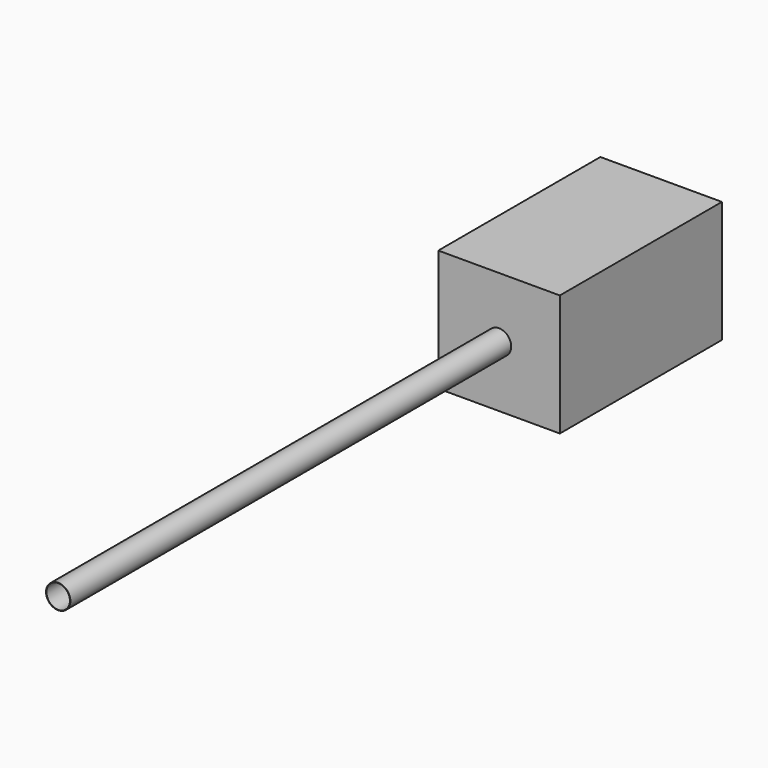
from build123d import *

# Parameters (mm, degrees)
F0_R          = 30
F1_DEPTH      = 1500
F2_R          = 29
F3_DEPTH      = 1500
F7_DEPTH      = 150
F7_DEPTH_BACK = 150


# Not quite as in the source:
# - the program builds the solid bodies; features that only make, move or delete a surface that nothing else refers to are left out


with BuildPart() as f1:
    # F0 (on Front) → F1 (new body)
    with BuildSketch(Plane.XZ):
        Circle(F0_R)
    extrude(amount=F1_DEPTH)

    # F2 (on face) → F3 (cut)
    with BuildSketch(Plane.XZ.offset(1500)):
        Circle(F2_R)
    extrude(amount=-F3_DEPTH, mode=Mode.SUBTRACT)

    # F6 (on Right) → F7 (join, two sides)
    with BuildSketch(Plane.YZ) as f7_sk:
        Polygon((-140, 150), (-140, 0), (-140, -150), (360, -150), (360, 150), align=None)
    extrude(amount=F7_DEPTH)
    extrude(f7_sk.sketch, amount=-F7_DEPTH_BACK)


solid = f1.part
